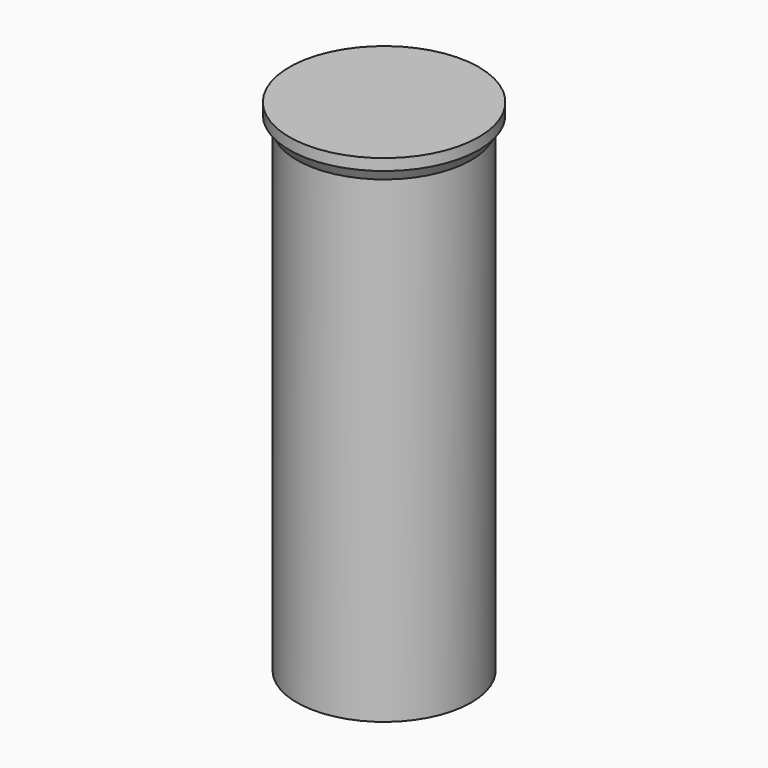
from build123d import *

# Parameters (mm, degrees)
F0_R     = 12.5
F1_DEPTH = 1.5
F3_DEPTH = 1.5
F4_DEPTH = 63


# Not quite as in the source:
# - a fillet or chamfer that OpenCascade refuses, or shapes differently, is made with other operations: its cross-section is extruded or revolved along the edge and cut away or added


with BuildPart() as f1:
    # F0 (on Top) → F1 (new body)
    with BuildSketch(Plane.XY):
        Circle(F0_R)
    extrude(amount=-F1_DEPTH)

    # F2: chamfer of 1 x 1.7320508076 on 1 edges, made by hand

    # F2_s1 → F2_t2 (revolve, cut)
    with BuildSketch(Plane.XZ):
        Polygon((12.5, 0.2320508076), (11.5, -1.5), (12.5, -1.5), align=None)
    revolve(axis=Axis((0, 0, -1.5), (0, 0, 1)), mode=Mode.SUBTRACT)

    # F0 (on Top) → F3 (join)
    with BuildSketch(Plane.XY):
        Circle(F0_R)
    extrude(amount=F3_DEPTH)

    # F4 (add): a face of the model
    f4_faces = [f1.faces().sort_by_distance(p)[0] for p in [
        (0, 0, -1.5),
    ]]
    extrude(f4_faces, amount=F4_DEPTH)


solid = f1.part
